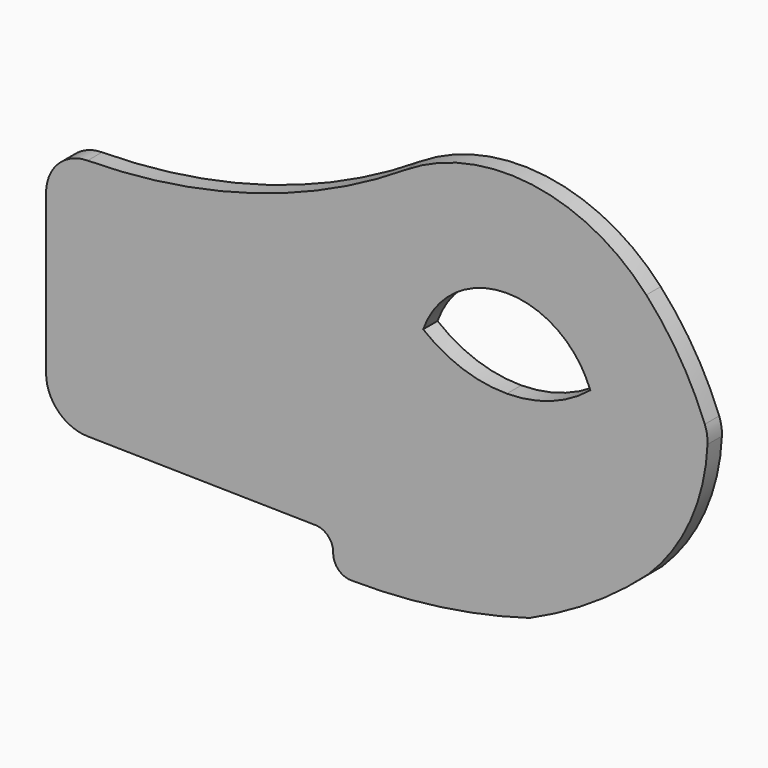
from build123d import *

# Parameters (mm, degrees)
F1_DEPTH = 3
F2_DEPTH = 25
F3_R     = 7
F4_R     = 100
F5_R     = 7
F6_R     = 3


# Not quite as in the source:
# - a feature names something its author has since deleted; it is built from what else it names


with BuildPart() as f1:
    # F0 (on Front) → F1 (new body)
    with BuildSketch(Plane.XZ):
        with BuildLine():
            Line((-28.5062876117, 71.7030383349), (-23.3711215756, 71.5975238881))
            ThreePointArc((-23.3711215756, 71.5975238881), (-24.6315082315, 75.5227380174), (-26.6928125912, 79.0930187933))
            ThreePointArc((-26.6928125912, 79.0930187933), (-46.4685424733, 86.625019162), (-61.3664115867, 71.5962461648))
            Line((-61.3664115867, 71.5962461648), (-56.3664115867, 71.5913571682))
            ThreePointArc((-56.3664115867, 71.5913571682), (-42.4756351566, 81.447422187), (-28.5062876117, 71.7030383349))
        make_face()
        with BuildLine():
            ThreePointArc((-61.3664115867, 71.5962461648), (-42.3681277411, 52.5998806027), (-23.3711215756, 71.5975238881))
            Line((-23.3711215756, 71.5975238881), (-28.5062876117, 71.7030383349))
            ThreePointArc((-28.5062876117, 71.7030383349), (-35.0280474509, 67.9936357913), (-42.4162418185, 66.6868830915))
            ThreePointArc((-42.4162418185, 66.6868830915), (-49.8149115034, 67.9342855664), (-56.3664115867, 71.5913571682))
            Line((-56.3664115867, 71.5913571682), (-61.3664115867, 71.5962461648))
        make_face()
        with BuildLine():
            ThreePointArc((-42.4162418185, 66.6868830915), (-35.0280474509, 67.9936357913), (-28.5062876117, 71.7030383349))
            ThreePointArc((-28.5062876117, 71.7030383349), (-42.4756351566, 81.447422187), (-56.3664115867, 71.5913571682))
            ThreePointArc((-56.3664115867, 71.5913571682), (-49.8149115034, 67.9342855664), (-42.4162418185, 66.6868830915))
        make_face()
        with BuildLine():
            Line((-20.8711215756, 71.5975236603), (-23.3711215756, 71.5975238881))
            ThreePointArc((-23.3711215756, 71.5975238881), (-42.3681277411, 52.5998806027), (-61.3664115867, 71.5962461648))
            Line((-61.3664115867, 71.5962461648), (-63.866411581, 71.5960777947))
            ThreePointArc((-63.866411581, 71.5960777947), (-63.6941147241, 68.8812286525), (-63.1803487139, 66.2098738354))
            ThreePointArc((-63.1803487139, 66.2098738354), (-48.9397473345, 51.1287456375), (-28.5819229469, 55.1029300277))
            ThreePointArc((-28.5819229469, 55.1029300277), (-22.8939959961, 62.4935676044), (-20.8711215756, 71.5975236602))
        make_face()
        with BuildLine():
            ThreePointArc((-26.6928125912, 79.0930187933), (-24.6315082315, 75.5227380174), (-23.3711215756, 71.5975238881))
            Line((-23.3711215756, 71.5975238881), (-20.8711215756, 71.5975236603))
            ThreePointArc((-20.8711215756, 71.5975236602), (-22.8939959961, 62.4935676044), (-28.5819229469, 55.1029300277))
            ThreePointArc((-28.5819229469, 55.1029300277), (-33.5715090435, 45.0303149316), (-38.6320985636, 34.9931849634))
            ThreePointArc((-38.6320985636, 34.9931849634), (-28.2353261857, 40.6242290748), (-18.8527258187, 47.819251244))
            ThreePointArc((-18.8527258187, 47.819251244), (-11.5073907557, 58.7139707043), (-8.9261215756, 71.5975225718))
            Line((-8.9261215756, 71.5975225718), (-11.6744206899, 71.5975225718))
            Line((-11.6744206899, 71.5975225718), (-11.6744206899, 74.0203762137))
            ThreePointArc((-11.6744206899, 74.0203762137), (-14.431706638, 81.8781100982), (-19.1607128583, 88.7325325952))
            ThreePointArc((-19.1607128583, 88.7325325952), (-48.5320541227, 98.3962580044), (-71.9061774941, 78.1548738354))
            Line((-71.9061774941, 78.1548738354), (-107.2845857728, 78.1548738354))
            Line((-107.2845857728, 78.1548738354), (-119.2295857724, 78.1548738354))
            Line((-119.2295857724, 78.1548738354), (-119.2295857724, 66.2098738355))
            Line((-119.2295857724, 66.2098738355), (-119.2295857724, 47.819251244))
            ThreePointArc((-119.2295857724, 47.819251244), (-113.3445755267, 44.456364285), (-107.2845857724, 41.4201036786))
            Line((-107.2845857724, 41.4201036786), (-107.2845857724, 66.2098738354))
            Line((-107.2845857724, 66.2098738354), (-68.5864427672, 66.2098738354))
            Line((-68.5864427672, 66.2098738354), (-63.1803487138, 66.2098738354))
            ThreePointArc((-63.1803487139, 66.2098738354), (-63.6941147241, 68.8812286525), (-63.866411581, 71.5960777947))
            Line((-63.866411581, 71.5960777947), (-61.3664115867, 71.5962461648))
            ThreePointArc((-61.3664115867, 71.5962461648), (-46.4685424733, 86.625019162), (-26.6928125912, 79.0930187933))
        make_face()
        with BuildLine():
            Line((-11.6744206899, 71.5975225718), (-8.9261215756, 71.5975225718))
            ThreePointArc((-8.9261215756, 71.5975225718), (-13.1797411051, 80.6808937542), (-19.1607128583, 88.7325325952))
            ThreePointArc((-19.1607128583, 88.7325325952), (-14.431706638, 81.8781100982), (-11.6744206899, 74.0203762137))
            Line((-11.6744206899, 74.0203762137), (-11.6744206899, 71.5975225718))
        make_face()
        with BuildLine():
            Line((-119.2295857724, 47.819251244), (-119.2295857724, 37.819251244))
            Line((-119.2295857724, 37.819251244), (-97.7339796794, 37.4339680289))
            ThreePointArc((-97.7339796794, 37.4339680289), (-102.5508909325, 39.3273444167), (-107.2845857724, 41.4201036786))
            ThreePointArc((-107.2845857724, 41.4201036786), (-113.3445755267, 44.456364285), (-119.2295857724, 47.819251244))
        make_face()
        with BuildLine():
            ThreePointArc((-38.6320985636, 34.9931849634), (-33.5715090435, 45.0303149316), (-28.5819229469, 55.1029300277))
            ThreePointArc((-28.5819229469, 55.1029300277), (-48.9397473345, 51.1287456375), (-63.1803487139, 66.2098738354))
            Line((-63.1803487138, 66.2098738354), (-68.5864427672, 66.2098738354))
            Line((-68.5864427672, 66.2098738354), (-107.2845857724, 66.2098738354))
            Line((-107.2845857724, 66.2098738354), (-107.2845857724, 41.4201036786))
            ThreePointArc((-107.2845857724, 41.4201036786), (-102.5508909325, 39.3273444167), (-97.7339796794, 37.4339680289))
            Line((-97.7339796794, 37.4339680289), (-71.3664115866, 36.9613606799))
            Line((-71.3664115866, 36.9613606799), (-71.3664115866, 30.923581687))
            ThreePointArc((-71.3664115866, 30.923581687), (-54.830296618, 31.5993469164), (-38.6320985636, 34.9931849634))
        make_face()
    extrude(amount=F1_DEPTH)

    # F0 (on Front) → F2 (cut)
    with BuildSketch(Plane.XZ):
        with BuildLine():
            ThreePointArc((-42.4162418185, 66.6868830915), (-35.0280474509, 67.9936357913), (-28.5062876117, 71.7030383349))
            ThreePointArc((-28.5062876117, 71.7030383349), (-42.4756351566, 81.447422187), (-56.3664115867, 71.5913571682))
            ThreePointArc((-56.3664115867, 71.5913571682), (-49.8149115034, 67.9342855664), (-42.4162418185, 66.6868830915))
        make_face()
    extrude(amount=F2_DEPTH, mode=Mode.SUBTRACT)

    # F3
    f3_edges = [f1.edges().sort_by_distance(p)[0] for p in [
        (-8.926122, -1.5, 71.597523),
        (-119.229586, -1.5, 37.819251),
    ]]
    fillet(f3_edges, radius=F3_R)

    # F4
    f4_edges = [f1.edges().sort_by_distance(p)[0] for p in [
        (-71.906177, -1.5, 78.154874),
    ]]
    fillet(f4_edges, radius=F4_R)

    # F5
    f5_edges = [f1.edges().sort_by_distance(p)[0] for p in [
        (-119.229586, -1.5, 78.154874),
    ]]
    fillet(f5_edges, radius=F5_R)

    # F6
    f6_edges = [f1.edges().sort_by_distance(p)[0] for p in [
        (-71.366412, -1.5, 36.961361),
        (-71.366412, -1.5, 30.923582),
    ]]
    fillet(f6_edges, radius=F6_R)


solid = f1.part
